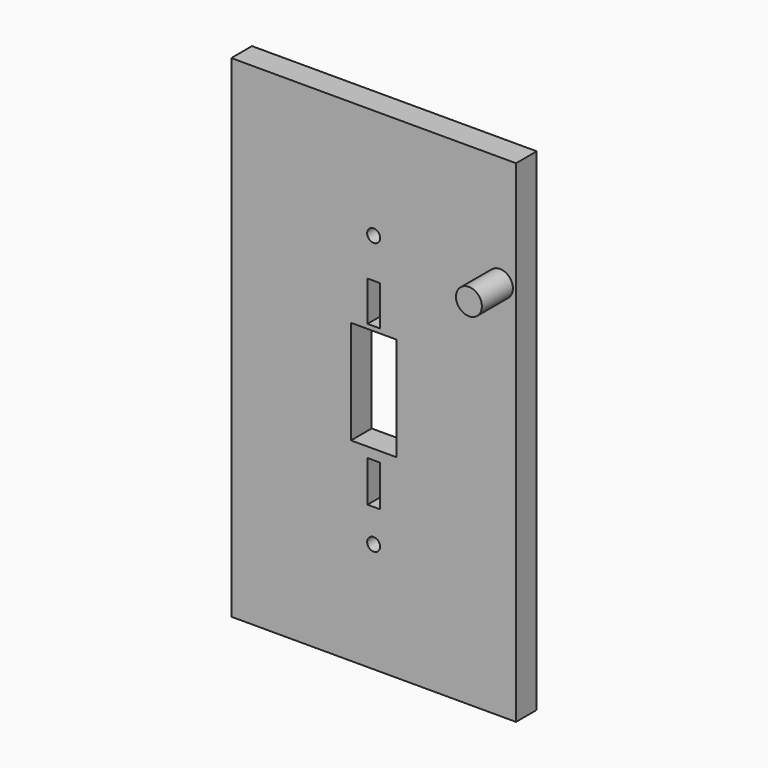
from build123d import *

# Parameters (mm, degrees)
F0_R     = 3.175
F1_DEPTH = 12.7
F0_W     = 69.85
F0_H     = 120.65
F0_R_2   = 1.5875
F0_W_2   = 3.0226
F0_H_2   = 1.0957790866
F0_H_3   = 2.4735292748
F2_DEPTH = 3.175


# Not quite as in the source:
# - a feature names something its author has since deleted; it is built from what else it names


with BuildPart() as f1:
    # F0 (on Front) → F1 (new body)
    with BuildSketch(Plane.XZ):
        with Locations((30.9913528, 33.0454)):
            Circle(F0_R)
    extrude(amount=F1_DEPTH)

    # F0 (on Front) → F2 (join, symmetric)
    with BuildSketch(Plane.XZ):
        Rectangle(F0_W, F0_H)
        with Locations((0, -33.3375)):
            Circle(F0_R_2, mode=Mode.SUBTRACT)
        Polygon((1.5113, 12.7), (5.55625, 12.7), (5.55625, -12.7), (1.5113, -12.7), (1.5113, -15.1735292748), (1.5113, -25.2650182862), (-1.5113, -25.2650182862), (-1.5113, -15.1735292748), (-1.5113, -12.7), (-5.55625, -12.7), (-5.55625, 12.7), (-1.5113, 12.7), (-1.5113, 13.7957790866), (-1.5113, 23.5874790866), (1.5113, 23.5874790866), (1.5113, 13.7957790866), align=None, mode=Mode.SUBTRACT)
        with Locations((0, 33.3375)):
            Circle(F0_R_2, mode=Mode.SUBTRACT)
        with Locations((30.9913528, 33.0454)):
            Circle(F0_R, mode=Mode.SUBTRACT)
        with Locations((0, 13.2478895433)):
            Rectangle(F0_W_2, F0_H_2)
        with Locations((30.9913528, 33.0454)):
            Circle(F0_R)
        with Locations((0, -13.9367646374)):
            Rectangle(F0_W_2, F0_H_3)
    extrude(amount=F2_DEPTH, both=True)


solid = f1.part
